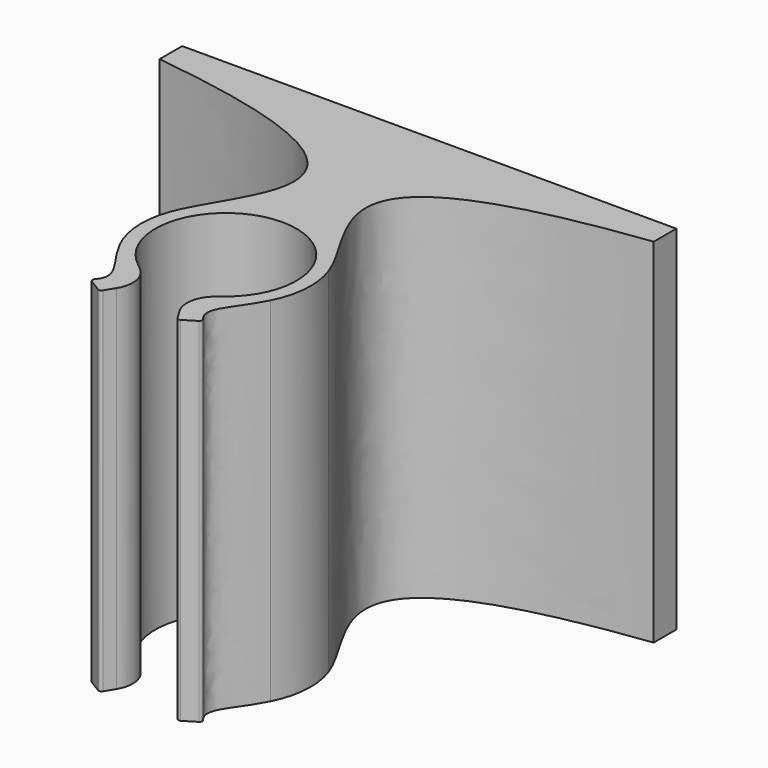
from build123d import *

# Parameters (mm, degrees)
F0_W        = 35
F0_H        = 2
F1_DEPTH    = 25
F2_T1_DEPTH = 33.357808199
F3_R        = 2


# Not quite as in the source:
# - a fillet or chamfer that OpenCascade refuses, or shapes differently, is made with other operations: its cross-section is extruded or revolved along the edge and cut away or added


with BuildPart() as f1:
    # F0 (on Top) → F1 (new body)
    with BuildSketch(Plane.XY):
        with Locations((0, 17)):
            Rectangle(F0_W, F0_H)
        with BuildLine():
            ThreePointArc((-5.6435050377, 2.0373637106), (0, 6), (5.6435050377, 2.0373637106))
            add(Edge.make_bspline(
                [(17.5, 16), (-4.7855940647, 13.2096234411), (3.9503478981, 6.7274152696), (5.6435050377, 2.0373637106)],
                knots=[0, 0, 0, 0, 18.317523985, 18.317523985, 18.317523985, 18.317523985], degree=3))
            Line((17.5, 16), (-17.5, 16))
            add(Edge.make_bspline(
                [(-17.5, 16), (4.7855940647, 13.2096234411), (-3.9503478981, 6.7274152696), (-5.6435050377, 2.0373637106)],
                knots=[0, 0, 0, 0, 18.317523985, 18.317523985, 18.317523985, 18.317523985], degree=3))
        make_face()
        with BuildLine():
            ThreePointArc((-1.5493444278, -4.7538964907), (0, 5), (1.5493444278, -4.7538964907))
            Line((1.5493444278, -4.7538964907), (1.5493444278, -5.7965103161))
            ThreePointArc((1.5493444278, -5.7965103161), (3.7756538243, -4.6630932007), (5.3474024613, -2.7212656829))
            ThreePointArc((5.3474024613, -2.7212656829), (5.9884180164, -0.3726253627), (5.6435050377, 2.0373637106))
            ThreePointArc((5.6435050377, 2.0373637106), (0, 6), (-5.6435050377, 2.0373637106))
            ThreePointArc((-5.6435050377, 2.0373637106), (-5.9884180164, -0.3726253627), (-5.3474024613, -2.7212656829))
            ThreePointArc((-5.3474024613, -2.7212656829), (-3.7756538243, -4.6630932007), (-1.5493444278, -5.7965103161))
            Line((-1.5493444278, -5.7965103161), (-1.5493444278, -4.7538964907))
        make_face()
        with BuildLine():
            Line((-2.6496251192, -7.5926648612), (-1.5493444278, -5.7965103161))
            ThreePointArc((-1.5493444278, -5.7965103161), (-3.7756538243, -4.6630932007), (-5.3474024613, -2.7212656829))
            add(Edge.make_bspline(
                [(-5.3474024613, -2.7212656829), (-4.3048003044, -4.7700231324), (-2.8869232094, -5.6816728311), (-3.8415154138, -6.828782889)],
                knots=[0, 0, 0, 0, 4.2754829053, 4.2754829053, 4.2754829053, 4.2754829053], degree=3))
            ThreePointArc((-3.8415154138, -6.828782889), (-3.8851139698, -6.989281561), (-3.7922551547, -7.1272594514))
            Line((-3.7922551547, -7.1272594514), (-2.9246420572, -7.6587381827))
            ThreePointArc((-2.9246420572, -7.6587381827), (-2.7734493553, -7.6826593947), (-2.6496251192, -7.5926648612))
        make_face()
        with BuildLine():
            ThreePointArc((5.3474024613, -2.7212656829), (3.7756538243, -4.6630932007), (1.5493444278, -5.7965103161))
            Line((1.5493444278, -5.7965103161), (2.6496251192, -7.5926648612))
            ThreePointArc((2.6496251192, -7.5926648612), (2.7734493553, -7.6826593947), (2.9246420572, -7.6587381827))
            Line((2.9246420572, -7.6587381827), (3.7922551547, -7.1272594514))
            ThreePointArc((3.7922551547, -7.1272594514), (3.8851139698, -6.989281561), (3.8415154138, -6.828782889))
            add(Edge.make_bspline(
                [(5.3474024613, -2.7212656829), (4.3048003044, -4.7700231324), (2.8869232094, -5.6816728311), (3.8415154138, -6.828782889)],
                knots=[0, 0, 0, 0, 4.2754829053, 4.2754829053, 4.2754829053, 4.2754829053], degree=3))
        make_face()
    extrude(amount=F1_DEPTH)

    # F2: fillet of radius 5 on 2 edges, made by hand

    # F2_s2 → F2_t1 (cut)
    with BuildSketch(Plane.XY.offset(-4.1789040995)):
        with BuildLine():
            ThreePointArc((-1.5493444278, -5.7965103161), (-2.1813631769, -4.7990149212), (-3.0296890274, -3.9775601061))
            ThreePointArc((-3.0296890274, -3.9775601061), (-2.3221889224, -4.4280287498), (-1.5493444278, -4.7538964907))
            Line((-1.5493444278, -4.7538964907), (-1.5493444278, -5.7965103161))
        make_face()
        with BuildLine():
            ThreePointArc((3.0296890274, -3.9775601061), (2.1813631769, -4.7990149212), (1.5493444278, -5.7965103161))
            Line((1.5493444278, -5.7965103161), (1.5493444278, -4.7538964907))
            ThreePointArc((1.5493444278, -4.7538964907), (2.3221889224, -4.4280287498), (3.0296890274, -3.9775601061))
        make_face()
    extrude(amount=F2_T1_DEPTH, mode=Mode.SUBTRACT)

    # F3
    f3_edges = [f1.edges().sort_by_distance(p)[0] for p in [
        (-1.549344, -5.79651, 12.5),
        (1.549344, -5.79651, 12.5),
    ]]
    fillet(f3_edges, radius=F3_R)


solid = f1.part
